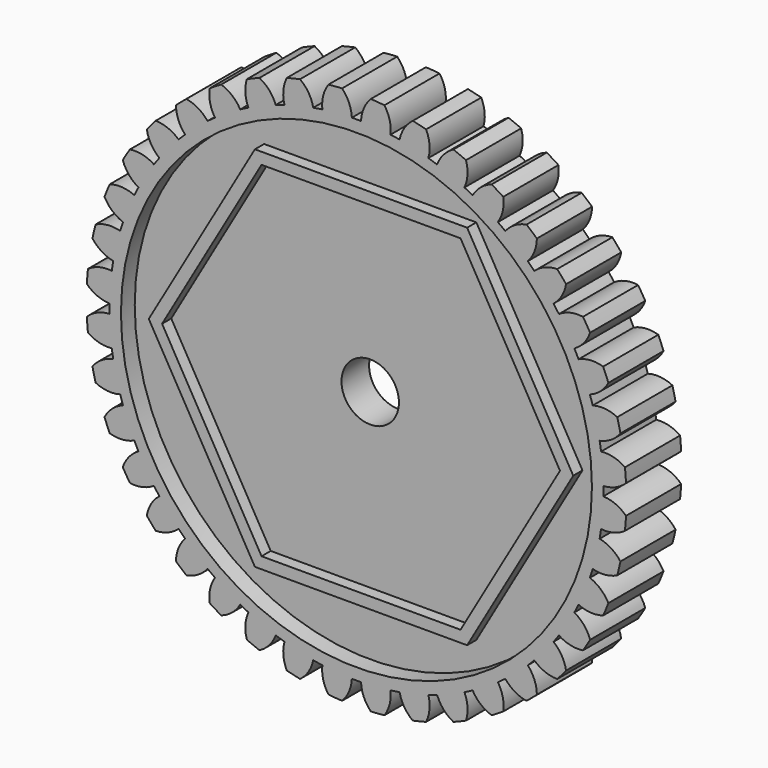
from build123d import *

# Parameters (mm, degrees)
F0_R            = 23.5
F0_R_2          = 2.5
F1_DEPTH        = 3
F1_DEPTH_BACK   = 3
F3_R            = 20.5
F4_DEPTH        = 1.5
F6_DEPTH        = 1
F8_DEPTH        = 3.001
F8_DEPTH_BACK   = 3.001
F8_COPIES_COUNT = 40


# Not quite as in the source:
# - a pattern or mirror of a feature is missing from the dataset's text; its kind, count and spacing are read off the source's solid


with BuildPart() as f1:
    # F0 (on Front) → F1 (new body, two sides)
    with BuildSketch(Plane.XZ) as f1_sk:
        Circle(F0_R)
        Circle(F0_R_2, mode=Mode.SUBTRACT)
    extrude(amount=F1_DEPTH)
    extrude(f1_sk.sketch, amount=-F1_DEPTH_BACK)

    # F3 (on face) → F4 (cut)
    with BuildSketch(Plane.XZ.offset(3)):
        Circle(F3_R)
    f4 = extrude(amount=-F4_DEPTH, mode=Mode.SUBTRACT)

    # F4_copies: F4 across plane
    add(f4.mirror(Plane.ZX), mode=Mode.SUBTRACT)

    # F5 (on face) → F6 (join)
    with BuildSketch(Plane.XZ.offset(1.5)):
        Polygon((-9.237604307, 16), (-18.4752086141, 0), (-9.237604307, -16), (9.237604307, -16), (18.4752086141, 0), (9.237604307, 16), align=None)
        Polygon((8.6602540378, 15), (17.3205080757, 0), (8.6602540378, -15), (-8.6602540378, -15), (-17.3205080757, 0), (-8.6602540378, 15), align=None, mode=Mode.SUBTRACT)
    f6 = extrude(amount=F6_DEPTH)

    # F6_copies: F6 across plane
    add(f6.mirror(Plane.ZX))

    # F7 (on Front) → F8 (cut, two sides)
    with BuildSketch(Plane.XZ) as f8_sk:
        with BuildLine():
            ThreePointArc((0, 21.5), (0.2000086546, 21.4990696668), (0.4, 21.4962787477))
            ThreePointArc((0.4, 21.4962787477), (0.6427845005, 22.5601080845), (1.25, 23.4667317707))
            ThreePointArc((1.25, 23.4667317707), (0, 23.5), (-1.25, 23.4667317707))
            ThreePointArc((-1.25, 23.4667317707), (-0.6427845005, 22.5601080845), (-0.4, 21.4962787477))
            ThreePointArc((-0.4, 21.4962787477), (-0.2000086546, 21.4990696668), (0, 21.5))
        make_face()
    f8 = extrude(amount=-F8_DEPTH, mode=Mode.SUBTRACT) + extrude(f8_sk.sketch, amount=F8_DEPTH_BACK, mode=Mode.SUBTRACT)

    # F8_copies: F8 ×40 about axis
    f8_copies_axis = Axis((0, 0, 0), (0, 1, 0))
    for i in range(1, F8_COPIES_COUNT):
        add(f8.rotate(f8_copies_axis, i * 360 / F8_COPIES_COUNT), mode=Mode.SUBTRACT)


solid = f1.part
